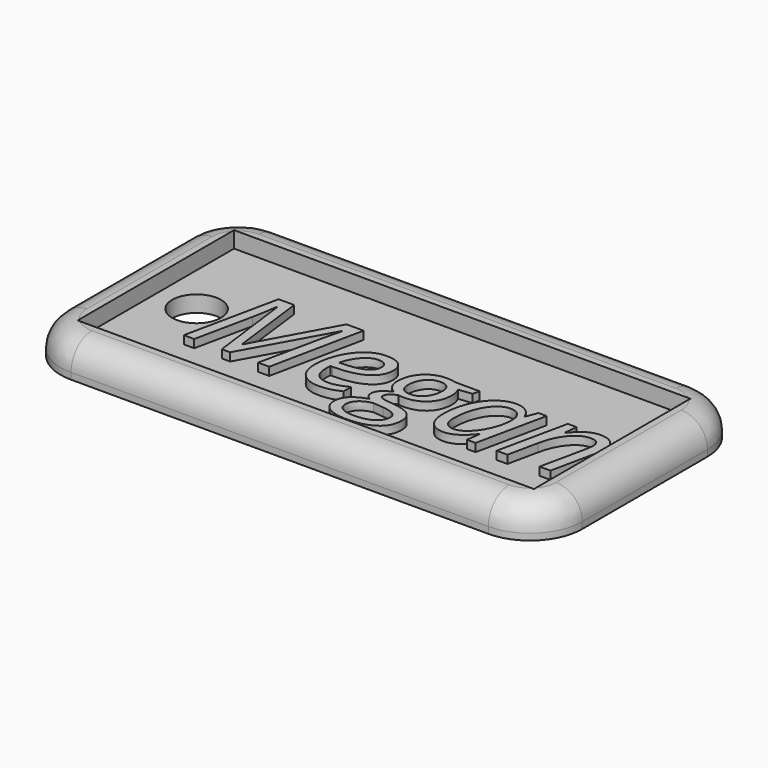
from build123d import *

# Parameters (mm, degrees)
F0_W         = 44.45
F0_H         = 19.05
F0_R         = 2.38125
F1_DEPTH     = 1.5875
F0_W_2       = 50.8
F0_H_2       = 25.4
F2_DEPTH     = 3.175
F3_R         = 5.08
F4_T1_DEPTH  = 40.64
F4_T3_DEPTH  = 15.24
F4_T6_ANGLE  = 90
F4_T8_ANGLE  = 90
F4_T10_ANGLE = 90
F4_T12_ANGLE = 90
F5_TEXT_SIZE = 12.781883944
F6_DEPTH     = 0.79375


# Not quite as in the source:
# - a fillet or chamfer that OpenCascade refuses, or shapes differently, is made with other operations: its cross-section is extruded or revolved along the edge and cut away or added
# - Text() gives the source's letters only with a copy of the font that has no kerning and outlines rounded to 1/6400 em; it was checked with that copy


with BuildPart() as f1:
    # F0 (on Top) → F1 (new body)
    with BuildSketch(Plane.XY):
        with Locations((25.4, 12.7)):
            Rectangle(F0_W, F0_H)
        with Locations((7.14375, 12.7)):
            Circle(F0_R, mode=Mode.SUBTRACT)
    extrude(amount=F1_DEPTH)

    # F0 (on Top) → F2 (join)
    with BuildSketch(Plane.XY):
        with Locations((25.4, 12.7)):
            Rectangle(F0_W_2, F0_H_2)
        with Locations((25.4, 12.7)):
            Rectangle(F0_W, F0_H, mode=Mode.SUBTRACT)
    extrude(amount=F2_DEPTH)

    # F3
    f3_edges = [f1.edges().sort_by_distance(p)[0] for p in [
        (0, 0, 1.5875),
        (50.8, 0, 1.5875),
        (50.8, 25.4, 1.5875),
        (0, 25.4, 1.5875),
    ]]
    fillet(f3_edges, radius=F3_R)

    # F4: fillet of radius 2.54 on 8 edges, made by hand

    # F4_s2 → F4_t1 (cut)
    with BuildSketch(Plane.YZ.offset(5.08)):
        with BuildLine():
            ThreePointArc((0, 0.635), (0.7439487758, 2.4310512242), (2.54, 3.175))
            Line((2.54, 3.175), (0, 3.175))
            Line((0, 3.175), (0, 0.635))
        make_face()
        with BuildLine():
            ThreePointArc((25.4, 0.635), (24.6560512242, 2.4310512242), (22.86, 3.175))
            Line((22.86, 3.175), (25.4, 3.175))
            Line((25.4, 3.175), (25.4, 0.635))
        make_face()
    extrude(amount=F4_T1_DEPTH, mode=Mode.SUBTRACT)

    # F4_s4 → F4_t3 (cut)
    with BuildSketch(Plane.XZ.offset(-20.32)):
        with BuildLine():
            ThreePointArc((0, 0.635), (0.7439487758, 2.4310512242), (2.54, 3.175))
            Line((2.54, 3.175), (0, 3.175))
            Line((0, 3.175), (0, 0.635))
        make_face()
        with BuildLine():
            ThreePointArc((50.8, 0.635), (50.0560512242, 2.4310512242), (48.26, 3.175))
            Line((48.26, 3.175), (50.8, 3.175))
            Line((50.8, 3.175), (50.8, 0.635))
        make_face()
    extrude(amount=F4_T3_DEPTH, mode=Mode.SUBTRACT)

    # F4_s5 → F4_t6 (revolve, cut)
    with BuildSketch(Plane.XZ.offset(-20.32)):
        with BuildLine():
            ThreePointArc((0, 0.635), (0.7439487758, 2.4310512242), (2.54, 3.175))
            Line((2.54, 3.175), (0, 3.175))
            Line((0, 3.175), (0, 0.635))
        make_face()
    revolve(axis=Axis((5.08, 20.32, 3.175), (0, 0, -1)), revolution_arc=F4_T6_ANGLE, mode=Mode.SUBTRACT)

    # F4_s7 → F4_t8 (revolve, cut)
    with BuildSketch(Plane.XZ.offset(-5.08)):
        with BuildLine():
            ThreePointArc((0, 0.635), (0.7439487758, 2.4310512242), (2.54, 3.175))
            Line((2.54, 3.175), (0, 3.175))
            Line((0, 3.175), (0, 0.635))
        make_face()
    revolve(axis=Axis((5.08, 5.08, 3.175), (0, 0, 1)), revolution_arc=F4_T8_ANGLE, mode=Mode.SUBTRACT)

    # F4_s9 → F4_t10 (revolve, cut)
    with BuildSketch(Plane.XZ.offset(-20.32)):
        with BuildLine():
            ThreePointArc((50.8, 0.635), (50.0560512242, 2.4310512242), (48.26, 3.175))
            Line((48.26, 3.175), (50.8, 3.175))
            Line((50.8, 3.175), (50.8, 0.635))
        make_face()
    revolve(axis=Axis((45.72, 20.32, 3.175), (0, 0, 1)), revolution_arc=F4_T10_ANGLE, mode=Mode.SUBTRACT)

    # F4_s11 → F4_t12 (revolve, cut)
    with BuildSketch(Plane.YZ.offset(45.72)):
        with BuildLine():
            ThreePointArc((0, 0.635), (0.7439487758, 2.4310512242), (2.54, 3.175))
            Line((2.54, 3.175), (0, 3.175))
            Line((0, 3.175), (0, 0.635))
        make_face()
    revolve(axis=Axis((45.72, 5.08, 3.175), (0, 0, 1)), revolution_arc=F4_T12_ANGLE, mode=Mode.SUBTRACT)

    # F5 (on face) → F6 (join)
    with BuildSketch(Plane.XY.offset(1.5875)):
        with Locations((9.525, 7.5165772978)):
            Text('Megan', F5_TEXT_SIZE, font='Open Sans', font_style=FontStyle.ITALIC, text_align=(TextAlign.LEFT, TextAlign.BOTTOM))
    extrude(amount=F6_DEPTH)


solid = f1.part
